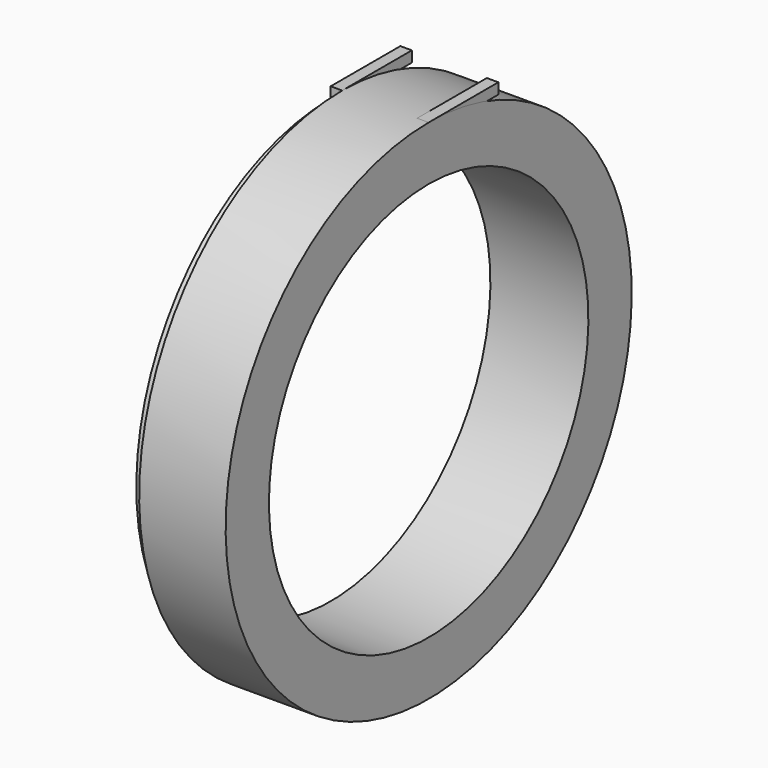
from build123d import *

# Parameters (mm, degrees)
F3_W     = 53.975
F3_H     = 408.7201654911
F4_DEPTH = 50.8


# Not quite as in the source:
# - the program builds the solid bodies; features that only make, move or delete a surface that nothing else refers to are left out


with BuildPart() as f4:
    # F3 (on face) → F4 (new body)
    with BuildSketch(Plane.XY.offset(-78.8711753155)):
        with Locations((-204.0980024693, 204.3600827456)):
            Rectangle(F3_W, F3_H)
    extrude(amount=-F4_DEPTH)


with BuildPart() as f4b:
    # F3 (on face) → F4, piece 2 (new body)
    with BuildSketch(Plane.XY.offset(-78.8711753155)):
        with Locations((201.8263277109, 204.3600827456)):
            Rectangle(F3_W, F3_H)
    extrude(amount=-F4_DEPTH)


with BuildPart() as f8:
    # F7 (on face) → F8 (revolve)
    with BuildSketch(Plane.XZ):
        Polygon((228.8138277109, -78.8711753155), (-177.1105024693, -78.8711753155), (-177.1105024693, -129.6711753155), (-231.0855024693, -129.6711753155), (-231.0855024693, -332.8711753155), (228.8138277109, -332.8711753155), align=None)
    revolve(axis=Axis((2.4814261124, 0, -1270), (-1, 0, 0)))


solid = Compound([f4.part, f4b.part, f8.part])
